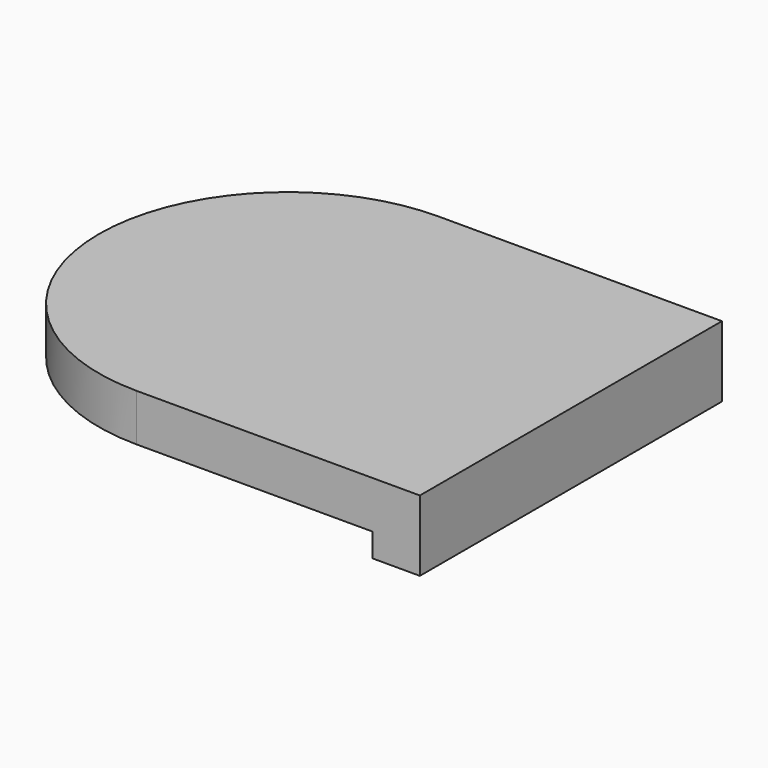
from build123d import *

# Parameters (mm, degrees)
F0_W     = 76.2
F0_H     = 101.6
F1_DEPTH = 19.05
F2_W     = 63.5
F2_H     = 6.35
F3_DEPTH = 164.846


with BuildPart() as f1:
    # F0 (on Top) → F1 (new body)
    with BuildSketch(Plane.XY):
        Rectangle(F0_W, F0_H)
        with BuildLine():
            ThreePointArc((-38.1, 50.8), (-88.9, 0), (-38.1, -50.8))
            Line((-38.1, -50.8), (-38.1, 50.8))
        make_face()
    extrude(amount=F1_DEPTH)

    # F2 (on face) → F3 (cut)
    with BuildSketch(Plane.XZ.offset(50.8)):
        with Locations((-6.35, 3.175)):
            Rectangle(F2_W, F2_H)
        Polygon((25.4, -12.1961906552), (25.4, 0), (-38.1, 0), (-38.1, 6.35), (-98.2422232628, 6.35), (-98.2422232628, -12.1961906552), align=None)
    extrude(amount=-F3_DEPTH, mode=Mode.SUBTRACT)


solid = f1.part
